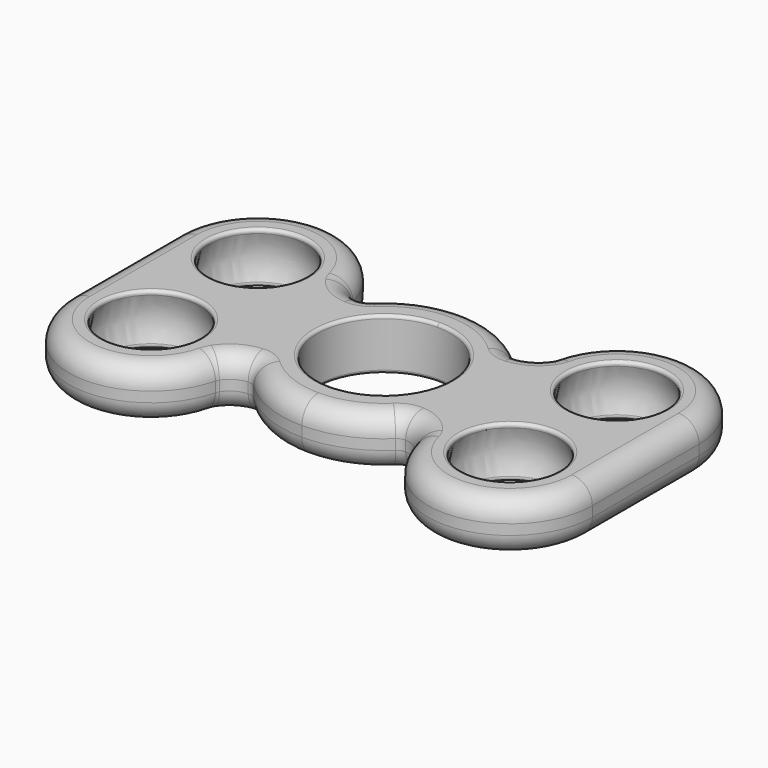
from build123d import *

# Parameters (mm, degrees)
F0_R     = 2.5
F1_DEPTH = 2.5
F2_DEPTH = 2.5
F11_R    = 2
F12_R    = 0.3


with BuildPart() as f1:
    # F0 (on Top) → F1 (new body)
    with BuildSketch(Plane.XY):
        with BuildLine():
            ThreePointArc((0, 6.525), (4.6138717472, 4.6138717472), (6.525, 0))
            ThreePointArc((6.525, 0), (4.6138717472, -4.6138717472), (0, -6.525))
            Line((0, -6.525), (0, -10))
            ThreePointArc((0, -10), (3.724907543, -9.2803590338), (6.9136958733, -7.2250127592))
            ThreePointArc((6.9136958733, -7.2250127592), (7.2653704993, -7.0069783722), (7.6752056708, -6.9499768925))
            ThreePointArc((7.6752056708, -6.9499768925), (8.7629642004, -7.2863778576), (9.5887267849, -8.0702786052))
            ThreePointArc((9.5887267849, -8.0702786052), (9.6704143129, -8.2213512626), (9.7250472259, -8.3841733891))
            ThreePointArc((9.7250472259, -8.3841733891), (18.4487828537, -14.4435389529), (25.5, -6.5))
            Line((25.5, -6.5), (25.5, 6.5))
            ThreePointArc((25.5, 6.5), (18.4487828537, 14.4435389529), (9.7250472259, 8.3841733891))
            ThreePointArc((9.7250472259, 8.3841733891), (9.6704143129, 8.2213512626), (9.5887267849, 8.0702786052))
            ThreePointArc((9.5887267849, 8.0702786052), (8.7629642004, 7.2863778576), (7.6752056708, 6.9499768925))
            ThreePointArc((7.6752056708, 6.9499768925), (7.2653704993, 7.0069783722), (6.9136958733, 7.2250127592))
            ThreePointArc((6.9136958733, 7.2250127592), (3.724907543, 9.2803590338), (0, 10))
            Line((0, 10), (0, 6.525))
        make_face()
        with Locations((17.5, -6.5)):
            Circle(F0_R, mode=Mode.SUBTRACT)
        with Locations((17.5, 6.5)):
            Circle(F0_R, mode=Mode.SUBTRACT)
        with BuildLine():
            ThreePointArc((0, -6.525), (-6.525, 0), (0, 6.525))
            Line((0, 6.525), (0, 10))
            ThreePointArc((0, 10), (-3.724907543, 9.2803590338), (-6.9136958733, 7.2250127592))
            ThreePointArc((-6.9136958733, 7.2250127592), (-7.2653704993, 7.0069783722), (-7.6752056708, 6.9499768925))
            ThreePointArc((-7.6752056708, 6.9499768925), (-8.7629642004, 7.2863778576), (-9.5887267849, 8.0702786052))
            ThreePointArc((-9.5887267849, 8.0702786052), (-9.6704143129, 8.2213512626), (-9.7250472259, 8.3841733891))
            ThreePointArc((-9.7250472259, 8.3841733891), (-18.4487828537, 14.4435389529), (-25.5, 6.5))
            Line((-25.5, 6.5), (-25.5, -6.5))
            ThreePointArc((-25.5, -6.5), (-18.4487828537, -14.4435389529), (-9.7250472259, -8.3841733891))
            ThreePointArc((-9.7250472259, -8.3841733891), (-9.6704143129, -8.2213512626), (-9.5887267849, -8.0702786052))
            ThreePointArc((-9.5887267849, -8.0702786052), (-8.7629642004, -7.2863778576), (-7.6752056708, -6.9499768925))
            ThreePointArc((-7.6752056708, -6.9499768925), (-7.2653704993, -7.0069783722), (-6.9136958733, -7.2250127592))
            ThreePointArc((-6.9136958733, -7.2250127592), (-3.724907543, -9.2803590338), (0, -10))
            Line((0, -10), (0, -6.525))
        make_face()
        with Locations((-17.5, -6.5)):
            Circle(F0_R, mode=Mode.SUBTRACT)
        with Locations((-17.5, 6.5)):
            Circle(F0_R, mode=Mode.SUBTRACT)
    extrude(amount=F1_DEPTH)

    # F0 (on Top) → F2 (join)
    with BuildSketch(Plane.XY):
        with BuildLine():
            ThreePointArc((0, 6.525), (4.6138717472, 4.6138717472), (6.525, 0))
            ThreePointArc((6.525, 0), (4.6138717472, -4.6138717472), (0, -6.525))
            Line((0, -6.525), (0, -10))
            ThreePointArc((0, -10), (3.724907543, -9.2803590338), (6.9136958733, -7.2250127592))
            ThreePointArc((6.9136958733, -7.2250127592), (7.2653704993, -7.0069783722), (7.6752056708, -6.9499768925))
            ThreePointArc((7.6752056708, -6.9499768925), (8.7629642004, -7.2863778576), (9.5887267849, -8.0702786052))
            ThreePointArc((9.5887267849, -8.0702786052), (9.6704143129, -8.2213512626), (9.7250472259, -8.3841733891))
            ThreePointArc((9.7250472259, -8.3841733891), (18.4487828537, -14.4435389529), (25.5, -6.5))
            Line((25.5, -6.5), (25.5, 6.5))
            ThreePointArc((25.5, 6.5), (18.4487828537, 14.4435389529), (9.7250472259, 8.3841733891))
            ThreePointArc((9.7250472259, 8.3841733891), (9.6704143129, 8.2213512626), (9.5887267849, 8.0702786052))
            ThreePointArc((9.5887267849, 8.0702786052), (8.7629642004, 7.2863778576), (7.6752056708, 6.9499768925))
            ThreePointArc((7.6752056708, 6.9499768925), (7.2653704993, 7.0069783722), (6.9136958733, 7.2250127592))
            ThreePointArc((6.9136958733, 7.2250127592), (3.724907543, 9.2803590338), (0, 10))
            Line((0, 10), (0, 6.525))
        make_face()
        with Locations((17.5, -6.5)):
            Circle(F0_R, mode=Mode.SUBTRACT)
        with Locations((17.5, 6.5)):
            Circle(F0_R, mode=Mode.SUBTRACT)
        with BuildLine():
            ThreePointArc((0, -6.525), (-6.525, 0), (0, 6.525))
            Line((0, 6.525), (0, 10))
            ThreePointArc((0, 10), (-3.724907543, 9.2803590338), (-6.9136958733, 7.2250127592))
            ThreePointArc((-6.9136958733, 7.2250127592), (-7.2653704993, 7.0069783722), (-7.6752056708, 6.9499768925))
            ThreePointArc((-7.6752056708, 6.9499768925), (-8.7629642004, 7.2863778576), (-9.5887267849, 8.0702786052))
            ThreePointArc((-9.5887267849, 8.0702786052), (-9.6704143129, 8.2213512626), (-9.7250472259, 8.3841733891))
            ThreePointArc((-9.7250472259, 8.3841733891), (-18.4487828537, 14.4435389529), (-25.5, 6.5))
            Line((-25.5, 6.5), (-25.5, -6.5))
            ThreePointArc((-25.5, -6.5), (-18.4487828537, -14.4435389529), (-9.7250472259, -8.3841733891))
            ThreePointArc((-9.7250472259, -8.3841733891), (-9.6704143129, -8.2213512626), (-9.5887267849, -8.0702786052))
            ThreePointArc((-9.5887267849, -8.0702786052), (-8.7629642004, -7.2863778576), (-7.6752056708, -6.9499768925))
            ThreePointArc((-7.6752056708, -6.9499768925), (-7.2653704993, -7.0069783722), (-6.9136958733, -7.2250127592))
            ThreePointArc((-6.9136958733, -7.2250127592), (-3.724907543, -9.2803590338), (0, -10))
            Line((0, -10), (0, -6.525))
        make_face()
        with Locations((-17.5, -6.5)):
            Circle(F0_R, mode=Mode.SUBTRACT)
        with Locations((-17.5, 6.5)):
            Circle(F0_R, mode=Mode.SUBTRACT)
    extrude(amount=-F2_DEPTH)

    # F3 (on Top) → F4 (revolve, cut)
    with BuildSketch(Plane.XY):
        with BuildLine():
            Line((-17.5, 1.27), (-17.5, 11.73))
            ThreePointArc((-17.5, 11.73), (-22.73, 6.5), (-17.5, 1.27))
        make_face()
    revolve(axis=Axis((-17.5, 6.5, 0), (0, -1, 0)), mode=Mode.SUBTRACT)

    # F5 (on Top) → F6 (revolve, cut)
    with BuildSketch(Plane.XY):
        with BuildLine():
            Line((-17.5, -11.73), (-17.5, -1.27))
            ThreePointArc((-17.5, -1.27), (-22.73, -6.5), (-17.5, -11.73))
        make_face()
    revolve(axis=Axis((-17.5, -6.5, 0), (0, -1, 0)), mode=Mode.SUBTRACT)

    # F7 (on Top) → F8 (revolve, cut)
    with BuildSketch(Plane.XY):
        with BuildLine():
            Line((17.5, 1.27), (17.5, 11.73))
            ThreePointArc((17.5, 11.73), (12.27, 6.5), (17.5, 1.27))
        make_face()
    revolve(axis=Axis((17.5, 6.5, 0), (0, -1, 0)), mode=Mode.SUBTRACT)

    # F9 (on Top) → F10 (revolve, cut)
    with BuildSketch(Plane.XY):
        with BuildLine():
            Line((17.5, -11.73), (17.5, -1.27))
            ThreePointArc((17.5, -1.27), (12.27, -6.5), (17.5, -11.73))
        make_face()
    revolve(axis=Axis((17.5, -6.5, 0), (0, -1, 0)), mode=Mode.SUBTRACT)

    # F11
    f11_edges = [f1.edges().sort_by_distance(p)[0] for p in [
        (0, 10, -2.5),
        (0, 10, 2.5),
    ]]
    fillet(f11_edges, radius=F11_R)

    # F12
    f12_edges = [f1.edges().sort_by_distance(p)[0] for p in [
        (-22.73, 6.5, 0),
        (-17.5, 11.093789, -2.5),
        (-17.5, 11.093789, 2.5),
        (-22.73, -6.5, 0),
        (-17.5, -1.906211, -2.5),
        (-17.5, -1.906211, 2.5),
        (6.525, 0, 1.25),
        (-6.525, 0, 0),
        (-6.525, 0, 2.5),
        (6.525, 0, -1.25),
        (-6.525, 0, -2.5),
        (12.27, 6.5, 0),
        (17.5, 11.093789, -2.5),
        (17.5, 11.093789, 2.5),
        (12.27, -6.5, 0),
        (17.5, -1.906211, -2.5),
        (17.5, -1.906211, 2.5),
    ]]
    fillet(f12_edges, radius=F12_R)


solid = f1.part
